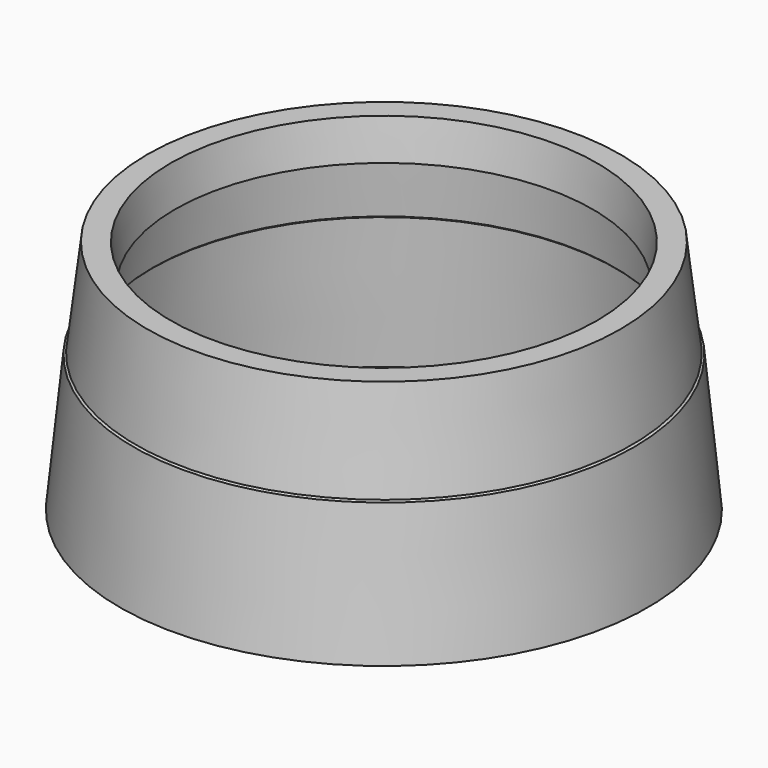
from build123d import *


with BuildPart() as f2:
    # F1 (on Front) → F2 (revolve)
    with BuildSketch(Plane.XZ):
        Polygon((-17.3, 17.26), (-18.15, 10.1), (-18.3, 10), (-19.3, 0), (-17.7, 0), (-17, 10), (-16.9, 10.1), (-16.471, 14.39), (-15.271, 14.39), (-15.59, 17.26), align=None)
    revolve(axis=Axis((0, 0, 5), (0, 0, 1)))


solid = f2.part
